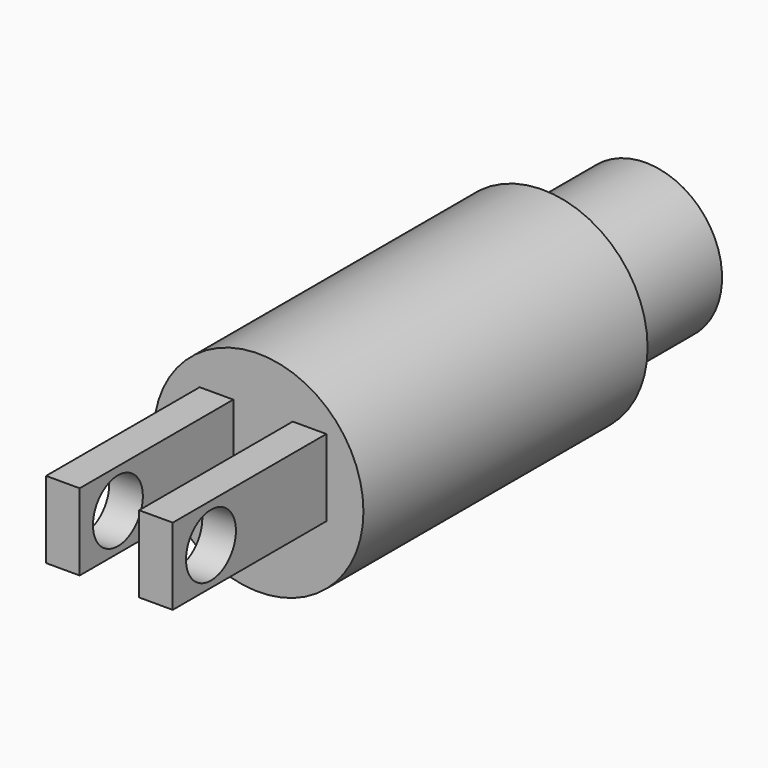
from build123d import *

# Parameters (mm, degrees)
F0_R     = 27.7491203527
F1_DEPTH = 93.98
F2_R     = 20.2221650078
F3_DEPTH = 34.036
F5_DEPTH = 50.8
F6_R     = 8.255
F8_DEPTH = 38.1


# Not quite as in the source:
# - the program builds the solid bodies; features that only make, move or delete a surface that nothing else refers to are left out


with BuildPart() as f1:
    # F0 (on Front) → F1 (new body)
    with BuildSketch(Plane.XZ):
        Circle(F0_R)
    extrude(amount=-F1_DEPTH)

    # F2 (on face) → F3 (join)
    with BuildSketch(Plane(origin=(0, 93.98, 0), x_dir=(-1, 0, 0), z_dir=(0, 1, 0))):
        Circle(F2_R)
    extrude(amount=F3_DEPTH)

    # F4 (on Front) → F5 (join)
    with BuildSketch(Plane.XZ):
        Polygon((-6.6853386185, -5.4466079127), (-6.6853386185, 0), (-6.6853386185, 14.8733920873), (-15.5753386185, 14.8733920873), (-15.5753386185, -5.4466079127), align=None)
        Polygon((9.04710629, 14.8733920873), (9.04710629, 0), (9.04710629, -5.4466079127), (17.93710629, -5.4466079127), (17.93710629, 14.8733920873), align=None)
    extrude(amount=F5_DEPTH)

    # F6 (on Right) → F8 (cut, symmetric)
    with BuildSketch(Plane.YZ):
        with Locations((-38.159750402, 4.5024077408)):
            Circle(F6_R)
    extrude(amount=F8_DEPTH, both=True, mode=Mode.SUBTRACT)


solid = f1.part
